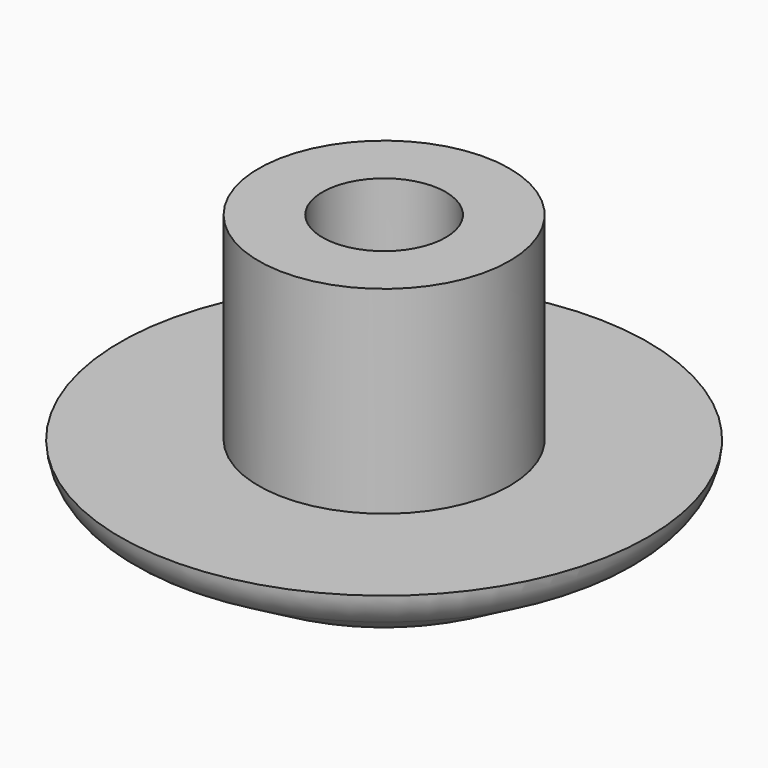
from build123d import *

# Parameters (mm, degrees)
F0_R     = 6
F1_DEPTH = 2
F2_SIZE2 = 2.5980762114
F2_SIZE  = 1.5
F4_R     = 2.85
F4_R_2   = 1.4
F5_DEPTH = 4.5
F6_R     = 1.2


# Not quite as in the source:
# - a fillet or chamfer that OpenCascade refuses, or shapes differently, is made with other operations: its cross-section is extruded or revolved along the edge and cut away or added


with BuildPart() as f1:
    # F0 (on Top) → F1 (new body)
    with BuildSketch(Plane.XY):
        Circle(F0_R)
    extrude(amount=F1_DEPTH)

    # F2
    f2_edges = [f1.edges().sort_by_distance(p)[0] for p in [
        (-6, 0, 0),
    ]]
    f2_side = f1.faces().sort_by_distance((-6, 0, 1))[0]
    chamfer(f2_edges, length=F2_SIZE, length2=F2_SIZE2, reference=f2_side)

    # F3: fillet of radius 1 on 2 edges, made by hand

    # F3_s1 → F3_t2 (revolve, cut)
    with BuildSketch(Plane.XZ):
        with BuildLine():
            ThreePointArc((3.6339745962, 0.1339745962), (3.3927936413, 0.0340741737), (3.1339745962, 0))
            Line((3.1339745962, 0), (3.4019237886, 0))
            Line((3.4019237886, 0), (3.6339745962, 0.1339745962))
        make_face()
    revolve(axis=Axis((0, 0, 0), (0, 0, 1)), mode=Mode.SUBTRACT)

    # F3_s3 → F3_t4 (revolve, cut)
    with BuildSketch(Plane.XZ):
        with BuildLine():
            ThreePointArc((6, 2), (5.8486778537, 1.5452494356), (5.5031382462, 1.2131367327))
            Line((5.5031382462, 1.2131367327), (6, 1.5))
            Line((6, 1.5), (6, 2))
        make_face()
    revolve(axis=Axis((0, 0, 1.5), (0, 0, 1)), mode=Mode.SUBTRACT)

    # F4 (on face) → F5 (join)
    with BuildSketch(Plane.XY.offset(2)):
        Circle(F4_R)
        Circle(F4_R_2, mode=Mode.SUBTRACT)
    extrude(amount=F5_DEPTH)

    # F6
    f6_edges = [f1.edges().sort_by_distance(p)[0] for p in [
        (-1.4, 0, 2),
    ]]
    fillet(f6_edges, radius=F6_R)


solid = f1.part
